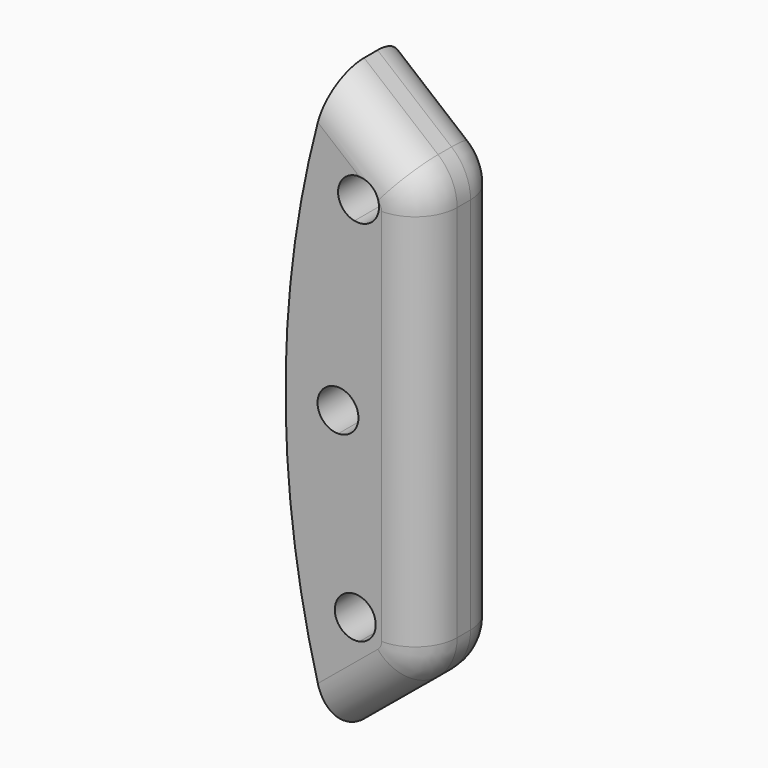
from build123d import *

# Parameters (mm, degrees)
F1_DEPTH     = 6.096
F3_DEPTH     = 25.4
F4_T1_DEPTH  = 45.8630415712
F4_T3_DEPTH  = 24.3228960689
F4_T5_DEPTH  = 24.3228960689
F4_T8_ANGLE  = 50.429603728
F4_T10_ANGLE = 50.429603728
F4_T12_ANGLE = 50.429603728
F4_T14_ANGLE = 50.429603728


# Not quite as in the source:
# - a fillet or chamfer that OpenCascade refuses, or shapes differently, is made with other operations: its cross-section is extruded or revolved along the edge and cut away or added


with BuildPart() as f1:
    # F0 (on Front) → F1 (new body, symmetric)
    with BuildSketch(Plane.XZ):
        with BuildLine():
            Line((0, -39.7012000674), (8.9594220974, -32.2971154711))
            ThreePointArc((8.9594220974, -32.2971154711), (10.6592614203, -30.1074484367), (11.2643083058, -27.4022656866))
            Line((11.2643083058, -27.4022656866), (11.2643083058, 18.4607758846))
            ThreePointArc((11.2643083058, 18.4607758846), (10.6592614203, 21.1659586348), (8.9594220974, 23.3556256691))
            Line((8.9594220974, 23.3556256691), (0, 30.7597102655))
            ThreePointArc((0, 30.7597102655), (-5.4521439637, -4.470744901), (0, -39.7012000674))
        make_face()
    extrude(amount=F1_DEPTH, both=True)

    # F2 (on face) → F3 (cut)
    with BuildSketch(Plane.XZ.offset(6.096)):
        with BuildLine():
            ThreePointArc((5.8633539044, 18.8184664851), (5.322886305, 20.3627562227), (3.9373851632, 21.2329990657))
            ThreePointArc((3.9373851632, 21.2329990657), (3.3868539044, 18.8184664851), (2.8907187579, 16.3921725692))
            ThreePointArc((2.8907187579, 16.3921725692), (4.9527998741, 16.8999083103), (5.8633539044, 18.8184664851))
        make_face()
        with BuildLine():
            ThreePointArc((5.4685295173, -25.8524299357), (4.5748708681, -23.9477867911), (2.5388582003, -23.4177455604))
            ThreePointArc((2.5388582003, -23.4177455604), (2.9920295173, -25.8524299357), (3.4997963379, -28.2763162998))
            ThreePointArc((3.4997963379, -28.2763162998), (4.9143376067, -27.4137703405), (5.4685295173, -25.8524299357))
        make_face()
        with BuildLine():
            ThreePointArc((3.4997963379, -28.2763162998), (2.9920295173, -25.8524299357), (2.5388582003, -23.4177455604))
            ThreePointArc((2.5388582003, -23.4177455604), (0.5625907808, -26.3329293377), (3.4997963379, -28.2763162998))
        make_face()
        with BuildLine():
            ThreePointArc((3.3743560218, -4.470744901), (2.6588166523, -2.7294609185), (0.9256825651, -1.9944012387))
            ThreePointArc((0.9256825651, -1.9944012387), (0.8978560218, -4.470744901), (0.9256825651, -6.9470885632))
            ThreePointArc((0.9256825651, -6.9470885632), (2.6588166523, -6.2120288835), (3.3743560218, -4.470744901))
        make_face()
        with BuildLine():
            ThreePointArc((0.9256825651, -6.9470885632), (0.8978560218, -4.470744901), (0.9256825651, -1.9944012387))
            ThreePointArc((0.9256825651, -1.9944012387), (-1.5786439782, -4.470744901), (0.9256825651, -6.9470885632))
        make_face()
        with BuildLine():
            ThreePointArc((2.8907187579, 16.3921725692), (3.3868539044, 18.8184664851), (3.9373851632, 21.2329990657))
            ThreePointArc((3.9373851632, 21.2329990657), (0.9662878494, 19.3418327271), (2.8907187579, 16.3921725692))
        make_face()
    extrude(amount=-F3_DEPTH, mode=Mode.SUBTRACT)

    # F4: fillet of radius 5.08 on 10 edges, made by hand

    # F4_s2 → F4_t1 (cut)
    with BuildSketch(Plane.XY.offset(-27.4022656866)):
        with BuildLine():
            ThreePointArc((6.1843083058, -6.096), (9.7764107542, -4.6081024484), (11.2643083058, -1.016))
            Line((11.2643083058, -1.016), (11.2643083058, -6.096))
            Line((11.2643083058, -6.096), (6.1843083058, -6.096))
        make_face()
        with BuildLine():
            ThreePointArc((6.1843083058, 6.096), (9.7764107542, 4.6081024484), (11.2643083058, 1.016))
            Line((11.2643083058, 1.016), (11.2643083058, 6.096))
            Line((11.2643083058, 6.096), (6.1843083058, 6.096))
        make_face()
    extrude(amount=F4_T1_DEPTH, mode=Mode.SUBTRACT)

    # F4_s4 → F4_t3 (cut)
    with BuildSketch(Plane(origin=(-29.284836754, 0, -24.2010485008), x_dir=(0, 1, 0), z_dir=(0.7708424857, 0, 0.637025794))):
        with BuildLine():
            ThreePointArc((1.016, -30.6033717472), (4.6081024484, -29.1154741956), (6.096, -25.5233717472))
            Line((6.096, -25.5233717472), (6.096, -30.6033717472))
            Line((6.096, -30.6033717472), (1.016, -30.6033717472))
        make_face()
        with BuildLine():
            ThreePointArc((-1.016, -30.6033717472), (-4.6081024484, -29.1154741956), (-6.096, -25.5233717472))
            Line((-6.096, -25.5233717472), (-6.096, -30.6033717472))
            Line((-6.096, -30.6033717472), (-1.016, -30.6033717472))
        make_face()
    extrude(amount=F4_T3_DEPTH, mode=Mode.SUBTRACT)

    # F4_s6 → F4_t5 (cut)
    with BuildSketch(Plane(origin=(-6.1450273998, 0, 5.078263109), x_dir=(0, 1, 0), z_dir=(-0.7708424857, 0, 0.637025794))):
        with BuildLine():
            ThreePointArc((6.096, -18.630891522), (4.6081024484, -22.2229939704), (1.016, -23.710891522))
            Line((1.016, -23.710891522), (6.096, -23.710891522))
            Line((6.096, -23.710891522), (6.096, -18.630891522))
        make_face()
        with BuildLine():
            ThreePointArc((-6.096, -18.630891522), (-4.6081024484, -22.2229939704), (-1.016, -23.710891522))
            Line((-1.016, -23.710891522), (-6.096, -23.710891522))
            Line((-6.096, -23.710891522), (-6.096, -18.630891522))
        make_face()
    extrude(amount=F4_T5_DEPTH, mode=Mode.SUBTRACT)

    # F4_s7 → F4_t8 (revolve, cut)
    with BuildSketch(Plane(origin=(-10.5357150876, 0, -8.7067363212), x_dir=(0, 1, 0), z_dir=(-0.7708424857, 0, -0.637025794))):
        with BuildLine():
            ThreePointArc((6.096, 25.5233717472), (4.6081024484, 29.1154741956), (1.016, 30.6033717472))
            Line((1.016, 30.6033717472), (6.096, 30.6033717472))
            Line((6.096, 30.6033717472), (6.096, 25.5233717472))
        make_face()
    revolve(axis=Axis((4.9143083058, 6.096, -27.4022656866), (0, -1, 0)), revolution_arc=F4_T8_ANGLE, mode=Mode.SUBTRACT)

    # F4_s9 → F4_t10 (revolve, cut)
    with BuildSketch(Plane.XY.offset(18.4607758846)):
        with BuildLine():
            ThreePointArc((6.1843083058, 6.096), (9.7764107542, 4.6081024484), (11.2643083058, 1.016))
            Line((11.2643083058, 1.016), (11.2643083058, 6.096))
            Line((11.2643083058, 6.096), (6.1843083058, 6.096))
        make_face()
    revolve(axis=Axis((4.9143083058, 6.096, 18.4607758846), (0, -1, 0)), revolution_arc=F4_T10_ANGLE, mode=Mode.SUBTRACT)

    # F4_s11 → F4_t12 (revolve, cut)
    with BuildSketch(Plane(origin=(-10.5357150876, 0, -8.7067363212), x_dir=(0, 1, 0), z_dir=(-0.7708424857, 0, -0.637025794))):
        with BuildLine():
            ThreePointArc((-1.016, 30.6033717472), (-4.6081024484, 29.1154741956), (-6.096, 25.5233717472))
            Line((-6.096, 25.5233717472), (-6.096, 30.6033717472))
            Line((-6.096, 30.6033717472), (-1.016, 30.6033717472))
        make_face()
    revolve(axis=Axis((4.9143083058, -6.096, -27.4022656866), (0, -1, 0)), revolution_arc=F4_T12_ANGLE, mode=Mode.SUBTRACT)

    # F4_s13 → F4_t14 (revolve, cut)
    with BuildSketch(Plane.XY.offset(18.4607758846)):
        with BuildLine():
            ThreePointArc((6.1843083058, -6.096), (9.7764107542, -4.6081024484), (11.2643083058, -1.016))
            Line((11.2643083058, -1.016), (11.2643083058, -6.096))
            Line((11.2643083058, -6.096), (6.1843083058, -6.096))
        make_face()
    revolve(axis=Axis((4.9143083058, -6.096, 18.4607758846), (0, -1, 0)), revolution_arc=F4_T14_ANGLE, mode=Mode.SUBTRACT)


solid = f1.part
